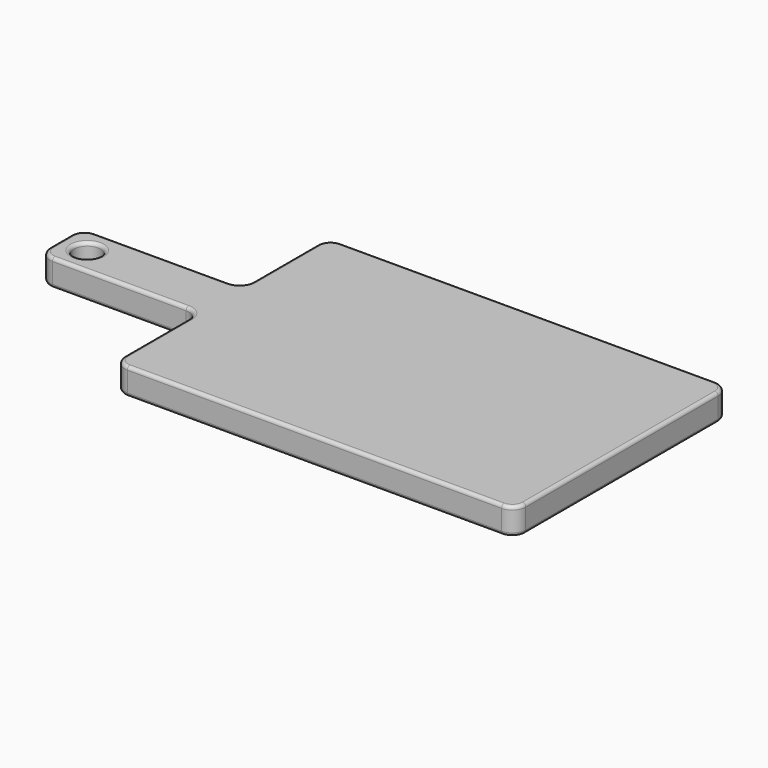
from build123d import *

# Parameters (mm, degrees)
F0_W         = 152.4
F0_H         = 50.8
F1_DEPTH     = 25.4
F2_R         = 12.7
F3_DEPTH     = 25.4
F1_FACE_R    = 12.7
F5_DEPTH     = 6.35
F6_R         = 6.35
F7_R         = 12.7
F8_R         = 3.175
F9_TEXT_SIZE = 44.9859991925
F10_DEPTH    = 0.508


# Not quite as in the source:
# - Text() gives the source's letters only with a copy of the font that has no kerning and outlines rounded to 1/6400 em; it was checked with that copy


with BuildPart() as f1:
    # F0 (on Top) → F1 (new body)
    with BuildSketch(Plane.XY):
        Polygon((0, 101.6), (0, 0), (381, 0), (381, 254), (0, 254), (0, 152.4), align=None)
        with Locations((-76.2, 127)):
            Rectangle(F0_W, F0_H)
    extrude(amount=F1_DEPTH)

    # F2 (on face) → F3 (cut)
    with BuildSketch(Plane.XY.offset(25.4)):
        with Locations((-127, 127)):
            Circle(F2_R)
    extrude(amount=-F3_DEPTH, mode=Mode.SUBTRACT)

    # F4 (on face) + F1_face (on face) → F5 (cut)
    with BuildSketch(Plane(origin=(0, 0, 0), x_dir=(1, 0, 0), z_dir=(0, 0, -1))):
        Polygon((12.7, -12.7), (12.7, -104.140000397), (12.7, -241.3), (368.3, -241.3), (368.3, -12.7), align=None)
        Polygon((355.5999953747, -228.5999953747), (25.4000046253, -228.5999953747), (25.4000046253, -104.140000397), (25.4000046253, -25.4000046253), (355.5999953747, -25.4000046253), align=None, mode=Mode.SUBTRACT)
    with BuildSketch(Plane(origin=(170.7444444444, 127, 25.4), x_dir=(1, 0, 0), z_dir=(0, 0, 1))):
        Polygon((-170.7444444444, -25.4), (-170.7444444444, -127), (210.2555555556, -127), (210.2555555556, 127), (-170.7444444444, 127), (-170.7444444444, 25.4), (-323.1444444444, 25.4), (-323.1444444444, -25.4), align=None)
        with Locations((-297.7444444444, 0)):
            Circle(F1_FACE_R, mode=Mode.SUBTRACT)
    extrude(amount=-F5_DEPTH, dir=(0, 0, -1), mode=Mode.SUBTRACT)

    # F6
    f6_edges = [f1.edges().sort_by_distance(p)[0] for p in [
        (12.7, 12.7, 3.175),
        (12.7, 241.3, 3.175),
        (368.3, 12.7, 3.175),
        (368.3, 241.3, 3.175),
    ]]
    fillet(f6_edges, radius=F6_R)

    # F7
    f7_edges = [f1.edges().sort_by_distance(p)[0] for p in [
        (0, 254, 12.7),
        (0, 0, 12.7),
        (381, 254, 12.7),
        (381, 0, 12.7),
        (-152.4, 152.4, 12.7),
        (-152.4, 101.6, 12.7),
        (0, 101.6, 12.7),
        (0, 152.4, 12.7),
    ]]
    fillet(f7_edges, radius=F7_R)

    # F8
    f8_edges = [f1.edges().sort_by_distance(p)[0] for p in [
        (25.400005, 127, 0),
        (190.5, 228.599995, 0),
        (355.599995, 127, 0),
        (190.5, 25.400005, 0),
        (0, 50.8, 0),
        (-3.719744, 97.880256, 0),
        (3.719744, 3.719744, 0),
        (-76.2, 101.6, 0),
        (190.5, 0, 0),
        (-148.680256, 105.319744, 0),
        (377.280256, 3.719744, 0),
        (-152.4, 127, 0),
        (381, 127, 0),
        (-148.680256, 148.680256, 0),
        (377.280256, 250.280256, 0),
        (-76.2, 152.4, 0),
        (190.5, 254, 0),
        (-3.719744, 156.119744, 0),
        (3.719744, 250.280256, 0),
        (0, 203.2, 0),
        (12.7, 127, 0),
        (14.559872, 239.440128, 0),
        (14.559872, 14.559872, 0),
        (190.5, 241.3, 0),
        (190.5, 12.7, 0),
        (366.440128, 239.440128, 0),
        (366.440128, 14.559872, 0),
        (368.3, 127, 0),
        (-139.7, 127, 0),
        (0, 50.8, 25.4),
        (-3.719744, 97.880256, 25.4),
        (3.719744, 3.719744, 25.4),
        (-76.2, 101.6, 25.4),
        (190.5, 0, 25.4),
        (-148.680256, 105.319744, 25.4),
        (377.280256, 3.719744, 25.4),
        (-152.4, 127, 25.4),
        (381, 127, 25.4),
        (-148.680256, 148.680256, 25.4),
        (377.280256, 250.280256, 25.4),
        (-76.2, 152.4, 25.4),
        (190.5, 254, 25.4),
        (-3.719744, 156.119744, 25.4),
        (3.719744, 250.280256, 25.4),
        (0, 203.2, 25.4),
        (-139.7, 127, 25.4),
    ]]
    fillet(f8_edges, radius=F8_R)

    # F9 (on face) → F10 (join)
    with BuildSketch(Plane(origin=(0, 0, 0), x_dir=(1, 0, 0), z_dir=(0, 0, -1))):
        with Locations((28.5750046253, -199.9792938294)):
            Text('Sophia Uecker', F9_TEXT_SIZE, font='Open Sans', font_style=FontStyle.BOLD, text_align=(TextAlign.LEFT, TextAlign.BOTTOM))
    extrude(amount=F10_DEPTH)


solid = f1.part
